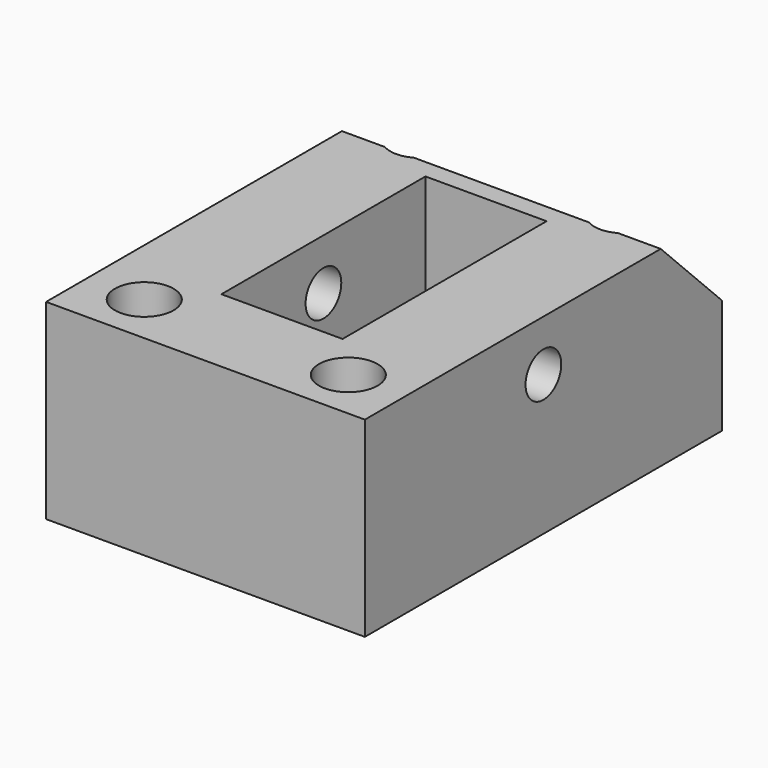
from build123d import *

# Parameters (mm, degrees)
F0_W         = 25
F0_H         = 35
F1_DEPTH     = 15
F2_R         = 1.75
F3_DEPTH     = 25
F4_W         = 9.5
F4_H         = 20
F5_DEPTH     = 15
F6_R         = 1.75
F7_DEPTH     = 4
F8_R         = 2.3
F9_DEPTH     = 15
F10_R        = 3
F10_R_2      = 2.3
F11_DEPTH    = 5
F12_T1_DEPTH = 55.8601958556


# Not quite as in the source:
# - a fillet or chamfer that OpenCascade refuses, or shapes differently, is made with other operations: its cross-section is extruded or revolved along the edge and cut away or added


with BuildPart() as f1:
    # F0 (on Top) → F1 (new body)
    with BuildSketch(Plane.XY):
        Rectangle(F0_W, F0_H)
    extrude(amount=-F1_DEPTH)

    # F2 (on face) → F3 (cut)
    with BuildSketch(Plane.YZ.offset(12.5)):
        with Locations((0, -4)):
            Circle(F2_R)
    extrude(amount=-F3_DEPTH, mode=Mode.SUBTRACT)

    # F4 (on face) → F5 (cut)
    with BuildSketch(Plane.XY):
        Rectangle(F4_W, F4_H)
    extrude(amount=-F5_DEPTH, mode=Mode.SUBTRACT)

    # F6 (on face) → F7 (cut)
    with BuildSketch(Plane(origin=(-12.5, 0, 0), x_dir=(0, -1, 0), z_dir=(-1, 0, 0))):
        Polygon((-2.8, -2.3834192463), (-2.8, -5.6165807537), (0, -7.2331615075), (2.8, -5.6165807537), (2.8, -2.3834192463), (0, -0.7668384925), align=None)
        with Locations((0, -4)):
            Circle(F6_R, mode=Mode.SUBTRACT)
    extrude(amount=-F7_DEPTH, mode=Mode.SUBTRACT)

    # F8 (on face) → F9 (cut)
    with BuildSketch(Plane.XY):
        with Locations((-8, 13.5)):
            Circle(F8_R)
        with Locations((8, 13.5)):
            Circle(F8_R)
        with Locations((8, -13.5)):
            Circle(F8_R)
        with Locations((-8, -13.5)):
            Circle(F8_R)
    extrude(amount=-F9_DEPTH, mode=Mode.SUBTRACT)

    # F10 (on face) → F11 (cut)
    with BuildSketch(Plane(origin=(0, 0, -15), x_dir=(1, 0, 0), z_dir=(0, 0, -1))):
        with Locations((-8, 13.5)):
            Circle(F10_R)
        with Locations((-8, 13.5)):
            Circle(F10_R_2, mode=Mode.SUBTRACT)
        with Locations((8, 13.5)):
            Circle(F10_R)
        with Locations((8, 13.5)):
            Circle(F10_R_2, mode=Mode.SUBTRACT)
        with Locations((8, -13.5)):
            Circle(F10_R)
        with Locations((8, -13.5)):
            Circle(F10_R_2, mode=Mode.SUBTRACT)
        with Locations((-8, -13.5)):
            Circle(F10_R)
        with Locations((-8, -13.5)):
            Circle(F10_R_2, mode=Mode.SUBTRACT)
    extrude(amount=-F11_DEPTH, mode=Mode.SUBTRACT)

    # F12: chamfer of 6 on 1 edges, made by hand

    # F12_s2 → F12_t1 (cut)
    with BuildSketch(Plane.YZ.offset(-27.9300979278)):
        Polygon((17.5, -6), (11.5, 0), (17.5, 0), align=None)
    extrude(amount=F12_T1_DEPTH, mode=Mode.SUBTRACT)


solid = f1.part
